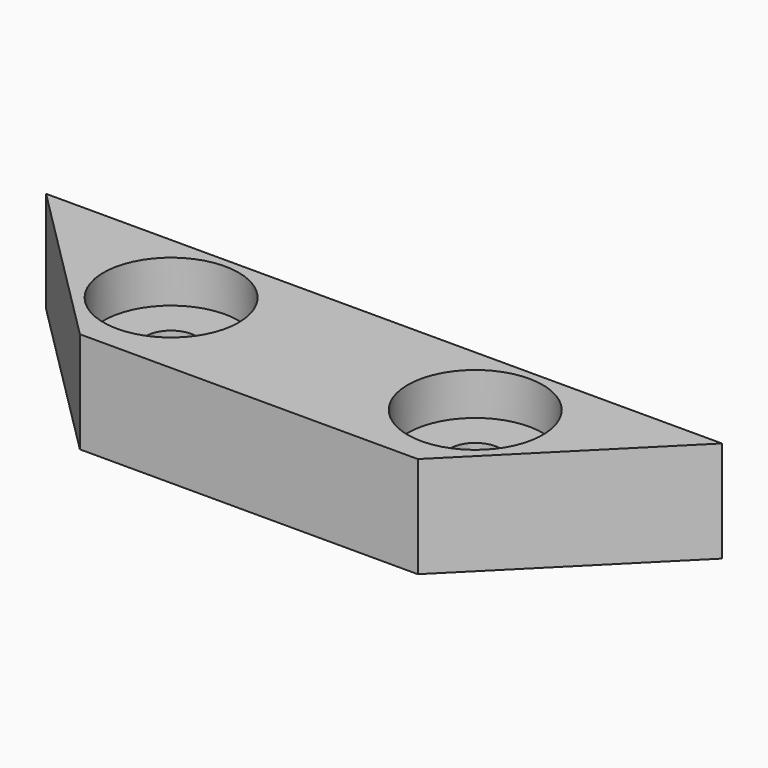
from build123d import *

# Parameters (mm, degrees)
F0_W           = 20
F0_H           = 10
F1_DEPTH       = 6
F2_SIZE        = 9.99999
F3_R           = 4
F4_DEPTH       = 2.5
F6_D           = 3
F6_DEPTH       = 10
F6_CBORE_D     = 3
F6_CBORE_DEPTH = 10
F6_TIP         = 0.9012909285


# Not quite as in the source:
# - a fillet or chamfer is up to 0.001 mm smaller than in the source, because OpenCascade refuses the exact size


with BuildPart() as f1:
    # F0 (on Top) → F1 (new body)
    with BuildSketch(Plane.XY):
        with Locations((-10, 0)):
            Rectangle(F0_W, F0_H)
    extrude(amount=F1_DEPTH)

    # F2 (size 10 in the source; OpenCascade refuses exactly that, so slightly less here)
    f2_edges = [f1.edges().sort_by_distance(p)[0] for p in [
        (-20, -5, 3),
    ]]
    chamfer(f2_edges, length=F2_SIZE)

    # F3 (on face) → F4 (cut)
    with BuildSketch(Plane.XY.offset(6)):
        with Locations((-9, 0.5)):
            Circle(F3_R)
    extrude(amount=-F4_DEPTH, mode=Mode.SUBTRACT)

    # F6
    with Locations(Plane.XY.offset(3.5)):
        with Locations((-9, 0.5)):
            CounterBoreHole(F6_D / 2, F6_CBORE_D / 2, F6_CBORE_DEPTH, depth=F6_DEPTH)
            with Locations((0, 0, -(F6_DEPTH + F6_TIP / 2))):  # 118° drill point
                Cone(0, F6_D / 2, F6_TIP, mode=Mode.SUBTRACT)

    # F7: F1 across plane


with BuildPart() as f1_1:
    add(f1.part)
    add(f1.part.mirror(Plane.YZ))


solid = f1_1.part
